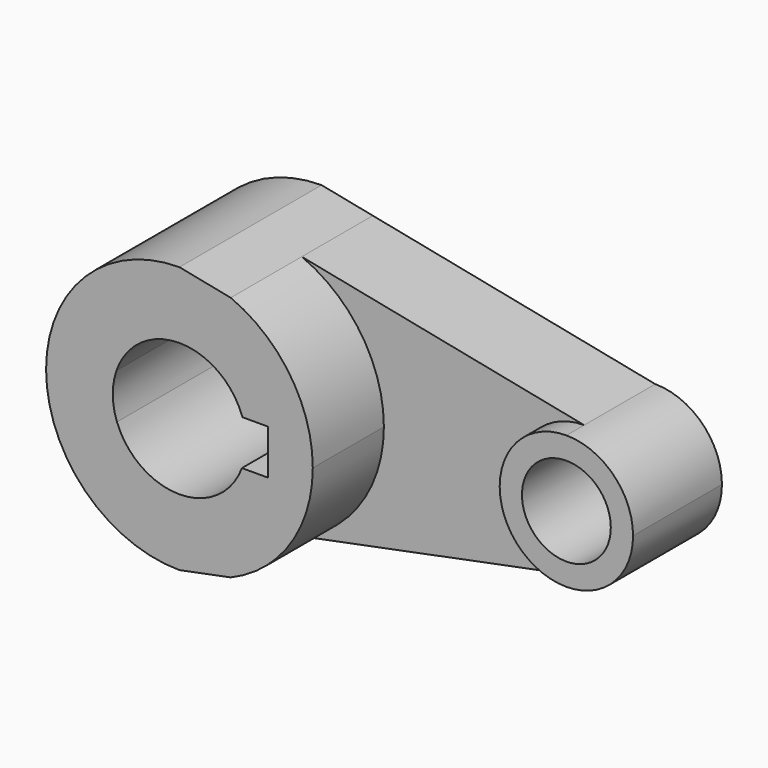
from build123d import *

# Parameters (mm, degrees)
F1_DEPTH = 50.8
F2_DEPTH = 25.4
F0_R     = 12.7
F3_DEPTH = 31.75


with BuildPart() as f1:
    # F0 (on Front) → F1 (new body)
    with BuildSketch(Plane.XZ):
        with BuildLine():
            Line((-23.4679372151, 35.1908475518), (-38.1188419469, 38.1188242326))
            ThreePointArc((-38.1188419469, 38.1188242326), (-76.2376661794, 0), (-38.1188419469, -38.1188242326))
            Line((-38.1188419469, -38.1188242326), (-23.4679372151, -35.1908475518))
            ThreePointArc((-23.4679372151, -35.1908475518), (-6.4051223354, -21.1491075291), (-1.77143e-05, 0))
            ThreePointArc((-1.77143e-05, 0), (-6.4051223354, 21.1491075291), (-23.4679372151, 35.1908475518))
        make_face()
        with BuildLine():
            ThreePointArc((-55.9794965989, -6.6256709397), (-57.1676480455, -0.2132749771), (-56.123365877, 6.2241158448))
            ThreePointArc((-56.123365877, 6.2241158448), (-38.1188419468, 19.05), (-20.1143180167, 6.2241158448))
            Line((-20.1143180167, 6.2241158448), (-12.8497872502, 6.2241158448))
            Line((-12.8497872502, 6.2241158448), (-12.8497872502, -6.6256709397))
            Line((-12.8497872502, -6.6256709397), (-20.2581872948, -6.6256709397))
            ThreePointArc((-20.2581872948, -6.6256709397), (-38.1188419468, -19.05), (-55.9794965989, -6.6256709397))
        make_face(mode=Mode.SUBTRACT)
    extrude(amount=F1_DEPTH)

    # F0 (on Front) → F2 (join)
    with BuildSketch(Plane.XZ):
        with BuildLine():
            Line((57.2499610198, 19.0594121163), (-23.4679372151, 35.1908475518))
            ThreePointArc((-23.4679372151, 35.1908475518), (-6.4051223354, 21.1491075291), (-1.77143e-05, 0))
            ThreePointArc((-1.77143e-05, 0), (-6.4051223354, -21.1491075291), (-23.4679372151, -35.1908475518))
            Line((-23.4679372151, -35.1908475518), (57.2499610198, -19.0594121163))
            ThreePointArc((57.2499610198, -19.0594121163), (38.1905489035, 0), (57.2499610198, 19.0594121163))
        make_face()
    extrude(amount=F2_DEPTH)

    # F0 (on Front) → F3 (join)
    with BuildSketch(Plane.XZ):
        with BuildLine():
            ThreePointArc((76.309373136, 0), (70.7270005726, 13.4770395529), (57.2499610198, 19.0594121163))
            ThreePointArc((57.2499610198, 19.0594121163), (38.1905489035, 0), (57.2499610198, -19.0594121163))
            ThreePointArc((57.2499610198, -19.0594121163), (70.7270005726, -13.4770395529), (76.309373136, 0))
        make_face()
        with Locations((57.2499610198, 0)):
            Circle(F0_R, mode=Mode.SUBTRACT)
    extrude(amount=F3_DEPTH)


solid = f1.part
